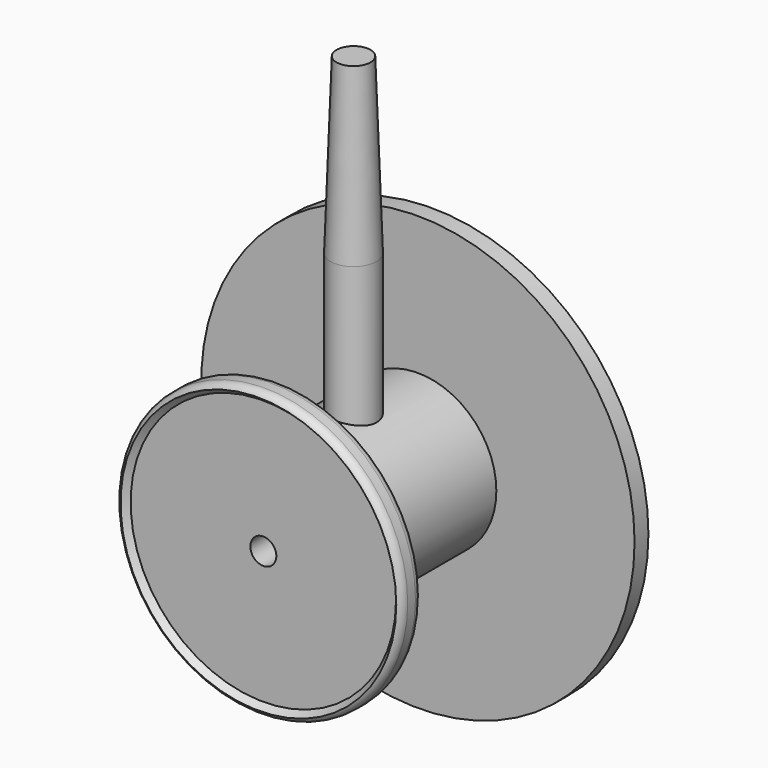
from build123d import *

# Parameters (mm, degrees)
F3_R     = 2.6577794355
F4_DEPTH = 45
F5_SIZE2 = 0.6984153898
F5_SIZE  = 20


# Not quite as in the source:
# - a fillet or chamfer that OpenCascade refuses, or shapes differently, is made with other operations: its cross-section is extruded or revolved along the edge and cut away or added


with BuildPart() as f1:
    # F0 (on Top) → F1 (revolve)
    with BuildSketch(Plane.XY):
        Polygon((25, 21.8126288628), (1.5, 21.8126288628), (1.5, -2.4768179283), (15.309067443, -2.4768179283), (15.9076526761, -3.1873711372), (16.5, -3.1873711372), (16.5, -0.1873711372), (9.0524229015, 0), (9.0524229015, 19.8126288628), (25, 19.8126288628), align=None)
    revolve(axis=Axis((0, 9.3126288628, 0), (0, 1, 0)))

    # F2: fillet of radius 1 on 2 edges, made by hand

    # F2_s1 → F2_t2 (revolve, cut)
    with BuildSketch(Plane.XY):
        with BuildLine():
            ThreePointArc((15.9076526761, -3.1873711372), (16.3389435845, -2.8184524698), (16.5, -2.2742340743))
            Line((16.5, -2.2742340743), (16.5, -3.1873711372))
            Line((16.5, -3.1873711372), (15.9076526761, -3.1873711372))
        make_face()
    revolve(axis=Axis((0, -3.1873711372, 0), (0, 1, 0)), mode=Mode.SUBTRACT)

    # F2_s3 → F2_t4 (revolve, cut)
    with BuildSketch(Plane.XY):
        with BuildLine():
            ThreePointArc((16.5, -1.1625288961), (16.2159436821, -0.4643708596), (15.5251507119, -0.1628452253))
            Line((15.5251507119, -0.1628452253), (16.5, -0.1873711372))
            Line((16.5, -0.1873711372), (16.5, -1.1625288961))
        make_face()
    revolve(axis=Axis((0, -0.1873711372, 0), (0, 1, 0)), mode=Mode.SUBTRACT)

    # F3 (on Top) → F4 (join)
    with BuildSketch(Plane.XY):
        with Locations((0, 10.5296224356)):
            Circle(F3_R)
    extrude(amount=F4_DEPTH)

    # F5
    f5_edges = [f1.edges().sort_by_distance(p)[0] for p in [
        (-2.657779, 10.529622, 45),
    ]]
    f5_side = f1.faces().sort_by_distance((-2.657779, 10.529622, 26.826736))[0]
    chamfer(f5_edges, length=F5_SIZE, length2=F5_SIZE2, reference=f5_side)


solid = f1.part
